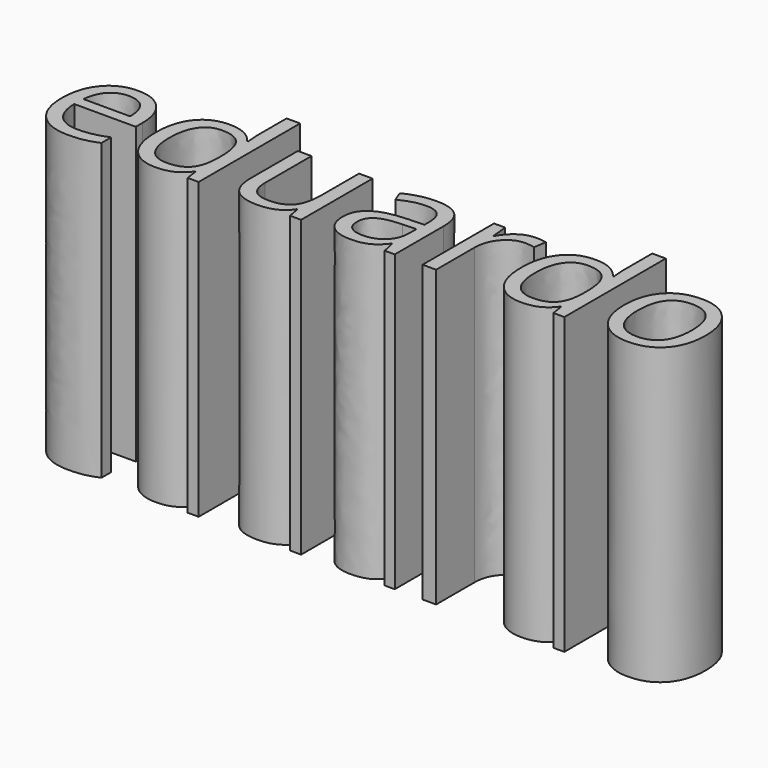
from build123d import *

# Parameters (mm, degrees)
F0_TEXT_SIZE = 14.3816384176
F1_DEPTH     = 25.4


# Not quite as in the source:
# - Text() gives the source's letters only with a copy of the font that has no kerning and outlines rounded to 1/6400 em; it was checked with that copy


with BuildPart() as f1:
    # F0 (on Top) → F1 (new body)
    with BuildSketch(Plane.XY):
        with Locations((-57.2029668062, -40.1834473014)):
            Text('eduardo', F0_TEXT_SIZE, font='Open Sans', text_align=(TextAlign.LEFT, TextAlign.BOTTOM))
    extrude(amount=F1_DEPTH)


solid = f1.part
